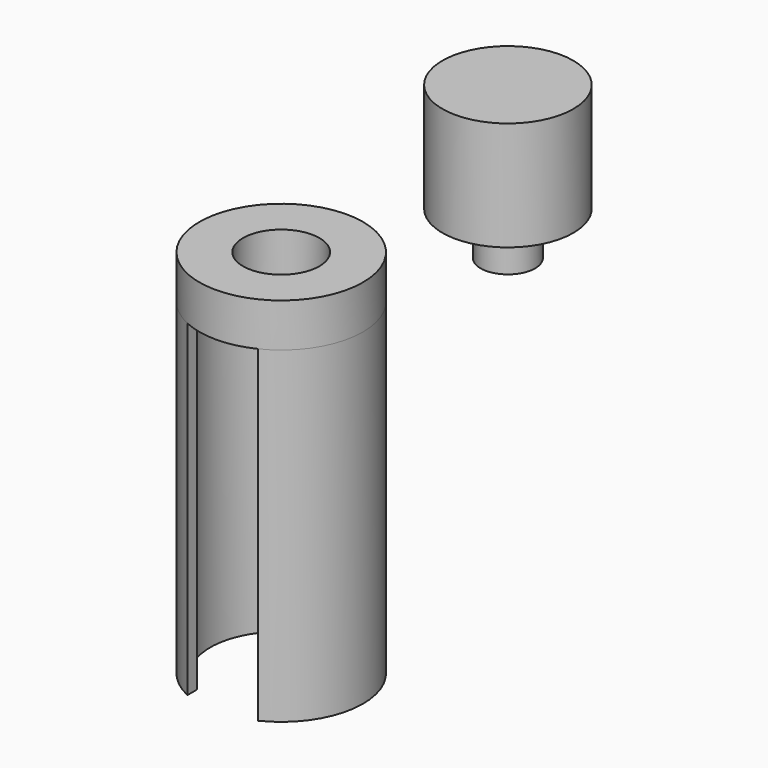
from build123d import *

# Parameters (mm, degrees)
F1_DEPTH = 30
F3_R     = 7.5
F3_R_2   = 3.5
F4_DEPTH = 4
F5_R     = 2.5
F5_R_2   = 2
F6_DEPTH = 4
F7_R     = 6
F8_DEPTH = 10


# Not quite as in the source:
# - a feature names something its author has since deleted; it is built from what else it names


with BuildPart() as f1:
    # F0 (on Top) → F1 (new body)
    with BuildSketch(Plane.XY):
        with BuildLine():
            Line((3.2850214823, -5.6087996809), (3.2781091996, -6.7456652804))
            ThreePointArc((3.2781091996, -6.7456652804), (-0.0698532595, 7.4996746944), (-3.1518908004, -6.8055554059))
            Line((-3.1518908004, -6.8055554059), (-3.1518908004, -5.684679796))
            ThreePointArc((-3.1518908004, -5.684679796), (-0.0766184872, 6.4995484157), (3.2850214823, -5.6087996809))
        make_face()
    extrude(amount=F1_DEPTH)

    # F3 (on offset) → F4 (join)
    with BuildSketch(Plane.XY.offset(30)):
        Circle(F3_R)
        Circle(F3_R_2, mode=Mode.SUBTRACT)
    extrude(amount=F4_DEPTH)


with BuildPart() as f6:
    # F5 (on offset) → F6 (new body)
    with BuildSketch(Plane.XY.offset(30)):
        with Locations((8.4675775911, 15.3844900672)):
            Circle(F5_R)
        with Locations((8.4675775911, 15.3844900672)):
            Circle(F5_R_2, mode=Mode.SUBTRACT)
    extrude(amount=F6_DEPTH)

    # F7 (on face) → F8 (join)
    with BuildSketch(Plane.XY.offset(34)):
        with Locations((8.4675775911, 15.3844900672)):
            Circle(F7_R)
    extrude(amount=F8_DEPTH)


solid = Compound([f1.part, f6.part])
